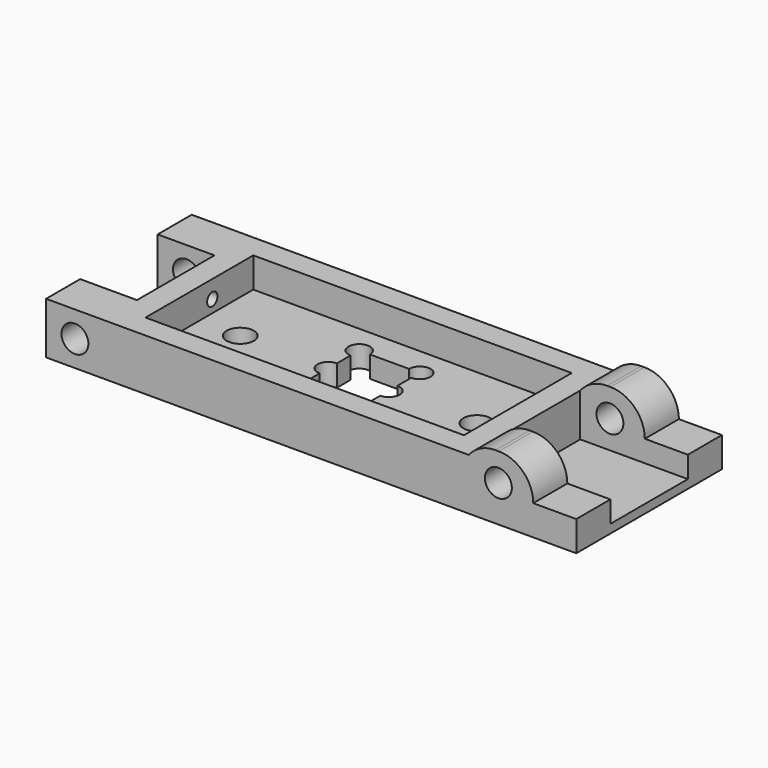
from build123d import *

# Parameters (mm, degrees)
F0_W         = 3.3528
F0_H         = 2.5146
F0_R         = 0.80645
F1_DEPTH     = 3.048
F2_W         = 2.54
F2_H         = 10.7442
F2_W_2       = 18.796
F2_H_2       = 7.9502
F3_DEPTH     = 1.27
F4_W         = 6.35
F4_H         = 5.715
F5_DEPTH     = 2.54
F6_R         = 0.79375
F7_DEPTH     = 10.7452
F8_DEPTH     = 0.508
F9_W         = 3.81
F9_H         = 2.5146
F10_DEPTH    = 0.762
F11_T1_DEPTH = 10.445747458
F11_T3_DEPTH = 10.445747458
F11_T5_DEPTH = 12.6746
F11_T7_DEPTH = 12.6746
F12_R        = 0.381
F8_FACE_W    = 7.9502
F8_FACE_H    = 1.778
F13_DEPTH    = 1.397


# Not quite as in the source:
# - a fillet or chamfer that OpenCascade refuses, or shapes differently, is made with other operations: its cross-section is extruded or revolved along the edge and cut away or added


with BuildPart() as f1:
    # F0 (on Top) → F1 (new body)
    with BuildSketch(Plane.XY):
        with Locations((-12.4714, 4.1148)):
            Rectangle(F0_W, F0_H)
        with Locations((-12.4714, -4.1148)):
            Rectangle(F0_W, F0_H)
        Polygon((10.795, 5.3721), (-10.795, 5.3721), (-10.795, 2.8575), (-10.795, -2.8575), (-10.795, -5.3721), (10.795, -5.3721), (17.145, -5.3721), (17.145, 5.3721), align=None)
        with Locations((-6.985, 0)):
            Circle(F0_R, mode=Mode.SUBTRACT)
        with BuildLine():
            ThreePointArc((-1.7885716042, 1.644670926), (-2.2375844102, 2.728683732), (-1.1535716042, 2.279670926))
            Line((-1.1535716042, 2.279670926), (1.1535716042, 2.279670926))
            ThreePointArc((1.1535716042, 2.279670926), (2.2375844102, 2.728683732), (1.7885716042, 1.644670926))
            Line((1.7885716042, 1.644670926), (1.7885716042, 0.635))
            ThreePointArc((1.7885716042, 0.635), (2.4235716042, 0), (1.7885716042, -0.635))
            Line((1.7885716042, -0.635), (1.7885716042, -1.644670926))
            ThreePointArc((1.7885716042, -1.644670926), (2.2375844102, -2.728683732), (1.1535716042, -2.279670926))
            Line((1.1535716042, -2.279670926), (-1.1535716042, -2.279670926))
            ThreePointArc((-1.1535716042, -2.279670926), (-2.2375844102, -2.728683732), (-1.7885716042, -1.644670926))
            Line((-1.7885716042, -1.644670926), (-1.7885716042, -0.635))
            ThreePointArc((-1.7885716042, -0.635), (-2.4235716042, 0), (-1.7885716042, 0.635))
            Line((-1.7885716042, 0.635), (-1.7885716042, 1.644670926))
        make_face(mode=Mode.SUBTRACT)
        with Locations((6.985, 0)):
            Circle(F0_R, mode=Mode.SUBTRACT)
    extrude(amount=F1_DEPTH)

    # F2 (on face) → F3 (cut)
    with BuildSketch(Plane.XY.offset(3.048)):
        with Locations((15.875, 0)):
            Rectangle(F2_W, F2_H)
        Rectangle(F2_W_2, F2_H_2)
    extrude(amount=-F3_DEPTH, mode=Mode.SUBTRACT)

    # F4 (on face) → F5 (cut)
    with BuildSketch(Plane.XY.offset(3.048)):
        with Locations((13.97, 0)):
            Rectangle(F4_W, F4_H)
    extrude(amount=-F5_DEPTH, mode=Mode.SUBTRACT)

    # F6 (on face) → F7 (cut, through all)
    with BuildSketch(Plane.XZ.offset(5.3721)):
        with Locations((-12.446, 1.524)):
            Circle(F6_R)
        with Locations((12.5476, 2.159)):
            Circle(F6_R)
    extrude(amount=-F7_DEPTH, mode=Mode.SUBTRACT)

    # F8 (cut): a face of the model
    f8_faces = [f1.faces().sort_by_distance(p)[0] for p in [
        (0, 3.7710178361, 1.778),
    ]]
    extrude(f8_faces, amount=-F8_DEPTH, mode=Mode.SUBTRACT)

    # F9 (on face) → F10 (join)
    with BuildSketch(Plane.XY.offset(3.048)):
        with Locations((12.7, 4.1148)):
            Rectangle(F9_W, F9_H)
        with Locations((12.7, -4.1148)):
            Rectangle(F9_W, F9_H)
    extrude(amount=F10_DEPTH)

    # F11: fillet of radius 2.032 on 4 edges, made by hand

    # F11_s2 → F11_t1 (cut)
    with BuildSketch(Plane.XZ.offset(-1.108073729)):
        with BuildLine():
            ThreePointArc((12.3812294916, 3.81), (11.5013476813, 3.6096200479), (10.795, 3.048))
            Line((10.795, 3.048), (10.795, 3.81))
            Line((10.795, 3.81), (12.3812294916, 3.81))
        make_face()
    extrude(amount=F11_T1_DEPTH, mode=Mode.SUBTRACT)

    # F11_s4 → F11_t3 (cut)
    with BuildSketch(Plane.XZ.offset(-9.337673729)):
        with BuildLine():
            ThreePointArc((12.3812294916, 3.81), (11.5013476813, 3.6096200479), (10.795, 3.048))
            Line((10.795, 3.048), (10.795, 3.81))
            Line((10.795, 3.81), (12.3812294916, 3.81))
        make_face()
    extrude(amount=F11_T3_DEPTH, mode=Mode.SUBTRACT)

    # F11_s6 → F11_t5 (cut)
    with BuildSketch(Plane.XZ.offset(-10.4521)):
        with BuildLine():
            ThreePointArc((14.605, 1.778), (14.0098409794, 3.2148409794), (12.573, 3.81))
            Line((12.573, 3.81), (14.605, 3.81))
            Line((14.605, 3.81), (14.605, 1.778))
        make_face()
    extrude(amount=F11_T5_DEPTH, mode=Mode.SUBTRACT)

    # F11_s8 → F11_t7 (cut)
    with BuildSketch(Plane.XZ.offset(-2.2225)):
        with BuildLine():
            ThreePointArc((14.605, 1.778), (14.0098409794, 3.2148409794), (12.573, 3.81))
            Line((12.573, 3.81), (14.605, 3.81))
            Line((14.605, 3.81), (14.605, 1.778))
        make_face()
    extrude(amount=F11_T7_DEPTH, mode=Mode.SUBTRACT)

    # F12 (on face) + F8_face (on face) → F13 (cut, through all)
    with BuildSketch(Plane(origin=(-10.795, 0, 0), x_dir=(0, -1, 0), z_dir=(-1, 0, 0))):
        with Locations((-0.9525, 2.0008196589)):
            Circle(F12_R)
    with BuildSketch(Plane(origin=(-9.398, 0, 2.159), x_dir=(0, 1, 0), z_dir=(1, 0, 0))):
        Rectangle(F8_FACE_W, F8_FACE_H)
    extrude(amount=-F13_DEPTH, dir=(-1, 0, 0), mode=Mode.SUBTRACT)


solid = f1.part
